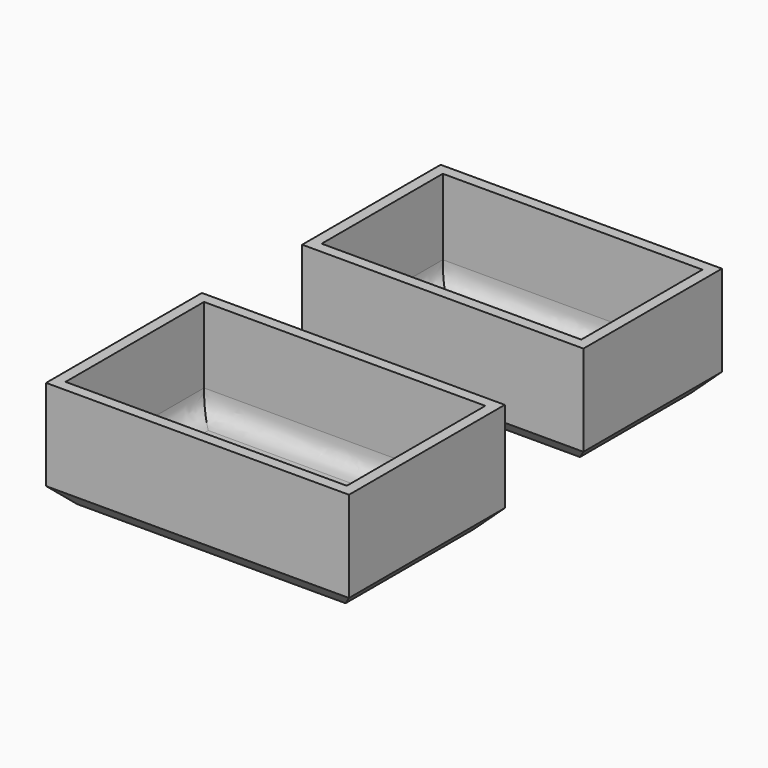
from build123d import *

# Parameters (mm, degrees)
F0_W        = 70
F0_H        = 45
F1_DEPTH    = 25
F2_T        = -2.5
F3_T1_DEPTH = 40
F3_T3_DEPTH = 65
F4_SIZE     = 4
F5_W        = 65
F5_H        = 40
F6_DEPTH    = 25
F7_T        = -2.5
F8_T1_DEPTH = 35
F8_T3_DEPTH = 60
F9_SIZE     = 4


# Not quite as in the source:
# - a fillet or chamfer that OpenCascade refuses, or shapes differently, is made with other operations: its cross-section is extruded or revolved along the edge and cut away or added


with BuildPart() as f1:
    # F0 (on Top) → F1 (new body)
    with BuildSketch(Plane.XY):
        with Locations((9.3095207959, -39.4999814034)):
            Rectangle(F0_W, F0_H)
    extrude(amount=F1_DEPTH)

    # F2
    f2_openings = [f1.faces().sort_by_distance(p)[0] for p in [
        (9.309521, -39.499981, 25),
    ]]
    offset(amount=F2_T, openings=f2_openings)

    # F3: fillet of radius 5 on 4 edges, made by hand

    # F3_s2 → F3_t1 (join)
    with BuildSketch(Plane.XZ.offset(19.4999814034)):
        with BuildLine():
            add(Edge.make_bspline(
                [(-23.1904792041, 7.5), (-23.1904792041, 2.5), (-18.1904792041, 2.5)],
                knots=[0, 0, 0, 1, 1, 1], degree=2, weights=[1, 1, 1]))
            Line((-18.1904792041, 2.5), (-23.1904792041, 2.5))
            Line((-23.1904792041, 2.5), (-23.1904792041, 7.5))
        make_face()
        with BuildLine():
            add(Edge.make_bspline(
                [(41.8095207959, 7.5), (41.8095207959, 2.5), (36.8095207959, 2.5)],
                knots=[0, 0, 0, 1, 1, 1], degree=2, weights=[1, 1, 1]))
            Line((36.8095207959, 2.5), (41.8095207959, 2.5))
            Line((41.8095207959, 2.5), (41.8095207959, 7.5))
        make_face()
    extrude(amount=F3_T1_DEPTH)

    # F3_s4 → F3_t3 (join)
    with BuildSketch(Plane.YZ.offset(-23.1904792041)):
        with BuildLine():
            add(Edge.make_bspline(
                [(-19.4999814034, 7.5), (-19.4999814034, 2.5), (-24.4999814034, 2.5)],
                knots=[0, 0, 0, 1, 1, 1], degree=2, weights=[1, 1, 1]))
            Line((-24.4999814034, 2.5), (-19.4999814034, 2.5))
            Line((-19.4999814034, 2.5), (-19.4999814034, 7.5))
        make_face()
        with BuildLine():
            add(Edge.make_bspline(
                [(-59.4999814034, 7.5), (-59.4999814034, 2.5), (-54.4999814034, 2.5)],
                knots=[0, 0, 0, 1, 1, 1], degree=2, weights=[1, 1, 1]))
            Line((-54.4999814034, 2.5), (-59.4999814034, 2.5))
            Line((-59.4999814034, 2.5), (-59.4999814034, 7.5))
        make_face()
    extrude(amount=F3_T3_DEPTH)

    # F4
    f4_edges = [f1.edges().sort_by_distance(p)[0] for p in [
        (9.309521, -61.999981, 0),
        (-25.690479, -39.499981, 0),
        (44.309521, -39.499981, 0),
        (9.309521, -16.999981, 0),
    ]]
    chamfer(f4_edges, length=F4_SIZE)


with BuildPart() as f6:
    # F5 (on Top) → F6 (new body)
    with BuildSketch(Plane.XY):
        with Locations((9.1597282141, 29.0331220999)):
            Rectangle(F5_W, F5_H)
    extrude(amount=F6_DEPTH)

    # F7
    f7_openings = [f6.faces().sort_by_distance(p)[0] for p in [
        (9.159728, 29.033122, 25),
    ]]
    offset(amount=F7_T, openings=f7_openings)

    # F8: fillet of radius 5 on 4 edges, made by hand

    # F8_s2 → F8_t1 (join)
    with BuildSketch(Plane.XZ.offset(-46.5331220999)):
        with BuildLine():
            add(Edge.make_bspline(
                [(-20.8402717859, 7.5), (-20.8402717859, 2.5), (-15.8402717859, 2.5)],
                knots=[0, 0, 0, 1, 1, 1], degree=2, weights=[1, 1, 1]))
            Line((-15.8402717859, 2.5), (-20.8402717859, 2.5))
            Line((-20.8402717859, 2.5), (-20.8402717859, 7.5))
        make_face()
        with BuildLine():
            add(Edge.make_bspline(
                [(39.1597282141, 7.5), (39.1597282141, 2.5), (34.1597282141, 2.5)],
                knots=[0, 0, 0, 1, 1, 1], degree=2, weights=[1, 1, 1]))
            Line((34.1597282141, 2.5), (39.1597282141, 2.5))
            Line((39.1597282141, 2.5), (39.1597282141, 7.5))
        make_face()
    extrude(amount=F8_T1_DEPTH)

    # F8_s4 → F8_t3 (join)
    with BuildSketch(Plane.YZ.offset(-20.8402717859)):
        with BuildLine():
            add(Edge.make_bspline(
                [(11.5331220999, 7.5), (11.5331220999, 2.5), (16.5331220999, 2.5)],
                knots=[0, 0, 0, 1, 1, 1], degree=2, weights=[1, 1, 1]))
            Line((16.5331220999, 2.5), (11.5331220999, 2.5))
            Line((11.5331220999, 2.5), (11.5331220999, 7.5))
        make_face()
        with BuildLine():
            add(Edge.make_bspline(
                [(46.5331220999, 7.5), (46.5331220999, 2.5), (41.5331220999, 2.5)],
                knots=[0, 0, 0, 1, 1, 1], degree=2, weights=[1, 1, 1]))
            Line((41.5331220999, 2.5), (46.5331220999, 2.5))
            Line((46.5331220999, 2.5), (46.5331220999, 7.5))
        make_face()
    extrude(amount=F8_T3_DEPTH)

    # F9
    f9_edges = [f6.edges().sort_by_distance(p)[0] for p in [
        (9.159728, 9.033122, 0),
        (-23.340272, 29.033122, 0),
        (9.159728, 49.033122, 0),
        (41.659728, 29.033122, 0),
    ]]
    chamfer(f9_edges, length=F9_SIZE)


solid = Compound([f1.part, f6.part])
